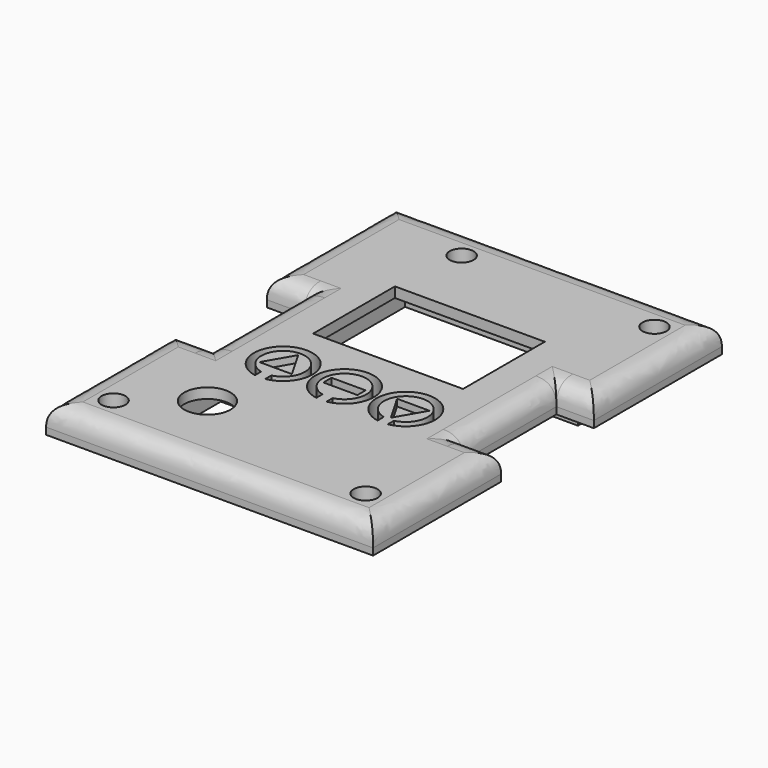
from build123d import *

# Parameters (mm, degrees)
F0_W          = 48
F0_H          = 64
F1_DEPTH      = 4
F2_W          = 5.5
F2_H          = 17
F3_DEPTH      = 4
F5_DEPTH      = 1.5
F6_R          = 1.05
F7_DEPTH      = 4
F8_W          = 22
F8_H          = 15
F9_DEPTH      = 5.501
F10_R         = 3.4
F11_DEPTH     = 5.501
F13_DEPTH     = 5.501
F14_W         = 14
F14_H         = 3.5
F15_DEPTH     = 4
F16_W         = 5
F16_H         = 1.5
F17_DEPTH     = 1
F19_DEPTH     = 4
F21_DEPTH     = 5
F22_T1_DEPTH  = 63
F22_T3_DEPTH  = 38.5
F22_T5_DEPTH  = 13
F22_T7_DEPTH  = 17
F22_T9_DEPTH  = 38.5
F22_T11_DEPTH = 13
F22_T17_DEPTH = 24.5
F22_T21_DEPTH = 20.5
F22_T28_DEPTH = 20.5
F22_T32_DEPTH = 24.5
F22_T39_DEPTH = 20.5
F22_T43_DEPTH = 24.5
F22_T50_DEPTH = 24.5
F22_T54_DEPTH = 20.5
F23_R         = 1.75
F24_DEPTH     = 3


# Not quite as in the source:
# - a fillet or chamfer that OpenCascade refuses, or shapes differently, is made with other operations: its cross-section is extruded or revolved along the edge and cut away or added
# - a feature names something its author has since deleted; it is built from what else it names


with BuildPart() as f1:
    # F0 (on Top) → F1 (new body)
    with BuildSketch(Plane.XY):
        Rectangle(F0_W, F0_H)
    extrude(amount=F1_DEPTH)

    # F2 (on face) → F3 (cut, through all)
    with BuildSketch(Plane(origin=(0, 0, 0), x_dir=(1, 0, 0), z_dir=(0, 0, -1))):
        with Locations((-21.25, 0)):
            Rectangle(F2_W, F2_H)
        with Locations((21.25, 0)):
            Rectangle(F2_W, F2_H)
    extrude(amount=-F3_DEPTH, mode=Mode.SUBTRACT)

    # F4 (on face) → F5 (join)
    with BuildSketch(Plane(origin=(0, 0, 0), x_dir=(1, 0, 0), z_dir=(0, 0, -1))):
        Polygon((-20.4, -10.1), (-20.4, -28.4), (-11.9, -28.4), (-11.9, -24.3), (-7.7, -24.3), (-7.7, -28.4), (16.3, -28.4), (16.3, -24.3), (20.4, -24.3), (20.4, -10.1), (15.5, -10.1), (15.5, 10.1), (20.4, 10.1), (20.4, 24.3), (16.3, 24.3), (16.3, 28.4), (-16.3, 28.4), (-16.3, 24.3), (-20.4, 24.3), (-20.4, 10.1), (-15.5, 10.1), (-15.5, -10.1), align=None)
    extrude(amount=F5_DEPTH)

    # F6 (on face) → F7 (cut, through all)
    with BuildSketch(Plane(origin=(0, 0, 0), x_dir=(1, 0, 0), z_dir=(0, 0, -1))):
        with Locations((-9.8, -26.5)):
            Circle(F6_R)
        with Locations((18.5, -26.5)):
            Circle(F6_R)
        with Locations((18.5, 26.5)):
            Circle(F6_R)
        with Locations((-18.5, 26.5)):
            Circle(F6_R)
    extrude(amount=-F7_DEPTH, mode=Mode.SUBTRACT)

    # F8 (on face) → F9 (cut, through all)
    with BuildSketch(Plane(origin=(0, 0, -1.5), x_dir=(1, 0, 0), z_dir=(0, 0, -1))):
        with Locations((0, -8.25)):
            Rectangle(F8_W, F8_H)
    extrude(amount=-F9_DEPTH, mode=Mode.SUBTRACT)

    # F10 (on face) → F11 (cut, through all)
    with BuildSketch(Plane(origin=(0, 0, -1.5), x_dir=(1, 0, 0), z_dir=(0, 0, -1))):
        with Locations((-10, 19.9)):
            Circle(F10_R)
    extrude(amount=-F11_DEPTH, mode=Mode.SUBTRACT)

    # F12 (on face) → F13 (cut, through all)
    with BuildSketch(Plane.XY.offset(4)):
        with BuildLine():
            ThreePointArc((0.75, -11.4840878593), (0, -2.95), (-0.75, -11.4840878593))
            Line((-0.75, -11.4840878593), (-0.75, -10.3608680461))
            ThreePointArc((-0.75, -10.3608680461), (0, -4.05), (0.75, -10.3608680461))
            Line((0.75, -10.3608680461), (0.75, -11.4840878593))
        make_face()
        with BuildLine():
            ThreePointArc((9.75, -11.4840878593), (9, -2.95), (8.25, -11.4840878593))
            Line((8.25, -11.4840878593), (8.25, -10.3608680461))
            ThreePointArc((8.25, -10.3608680461), (9, -4.05), (9.75, -10.3608680461))
            Line((9.75, -10.3608680461), (9.75, -11.4840878593))
        make_face()
        with BuildLine():
            ThreePointArc((-8.25, -11.4840878593), (-9, -2.95), (-9.75, -11.4840878593))
            Line((-9.75, -11.4840878593), (-9.75, -10.3608680461))
            ThreePointArc((-9.75, -10.3608680461), (-9, -4.05), (-8.25, -10.3608680461))
            Line((-8.25, -10.3608680461), (-8.25, -11.4840878593))
        make_face()
    extrude(amount=-F13_DEPTH, mode=Mode.SUBTRACT)

    # F14 (on face) → F15 (cut)
    with BuildSketch(Plane(origin=(0, 0, -1.5), x_dir=(1, 0, 0), z_dir=(0, 0, -1))):
        Polygon((-7, -0.75), (-13.5, -0.75), (-13.5, -20.75), (13.5, -20.75), (13.5, -0.75), (7, -0.75), align=None)
        with Locations((0, 1)):
            Rectangle(F14_W, F14_H)
    extrude(amount=-F15_DEPTH, mode=Mode.SUBTRACT)

    # F16 (on face) → F17 (cut)
    with BuildSketch(Plane.XY.offset(4)):
        Polygon((11.3815698604, -5.875), (6.6184301396, -5.875), (9, -10), align=None)
        Polygon((-9, -4.5), (-11.3815698604, -8.625), (-6.6184301396, -8.625), align=None)
        with Locations((0, -7.25)):
            Rectangle(F16_W, F16_H)
    extrude(amount=-F17_DEPTH, mode=Mode.SUBTRACT)

    # F18 (on face) → F19 (cut)
    with BuildSketch(Plane(origin=(0, 0, -1.5), x_dir=(1, 0, 0), z_dir=(0, 0, -1))):
        with BuildLine():
            ThreePointArc((-11.4264171117, 10.8), (-11.0070384176, 3.4471330828), (-4.7, 7.25))
            ThreePointArc((-4.7, 7.25), (-5.1971330828, 9.2570384176), (-6.5735828883, 10.8))
            Line((-6.5735828883, 10.8), (-11.4264171117, 10.8))
        make_face()
        with BuildLine():
            Line((-11.4264171117, 10.8), (-6.5735828883, 10.8))
            ThreePointArc((-6.5735828883, 10.8), (-9, 11.55), (-11.4264171117, 10.8))
        make_face()
        with BuildLine():
            ThreePointArc((-11.4264171117, 10.8), (-9, 11.55), (-6.5735828883, 10.8))
            Line((-6.5735828883, 10.8), (-2.4264171117, 10.8))
            ThreePointArc((-2.4264171117, 10.8), (0, 11.55), (2.4264171117, 10.8))
            Line((2.4264171117, 10.8), (6.5735828883, 10.8))
            ThreePointArc((6.5735828883, 10.8), (9, 11.55), (11.4264171117, 10.8))
            Line((11.4264171117, 10.8), (15.2, 10.8))
            Line((15.2, 10.8), (15.2, 26.3))
            Line((15.2, 26.3), (-15.3, 26.3))
            Line((-15.3, 26.3), (-15.3, 10.8))
            Line((-15.3, 10.8), (-11.4264171117, 10.8))
        make_face()
        with BuildLine():
            Line((2.4264171117, 10.8), (-2.4264171117, 10.8))
            ThreePointArc((-2.4264171117, 10.8), (-2.0070384176, 3.4471330828), (4.3, 7.25))
            ThreePointArc((4.3, 7.25), (3.8028669172, 9.2570384176), (2.4264171117, 10.8))
        make_face()
        with BuildLine():
            ThreePointArc((2.4264171117, 10.8), (0, 11.55), (-2.4264171117, 10.8))
            Line((-2.4264171117, 10.8), (2.4264171117, 10.8))
        make_face()
        with BuildLine():
            Line((11.4264171117, 10.8), (6.5735828883, 10.8))
            ThreePointArc((6.5735828883, 10.8), (6.9929615824, 3.4471330828), (13.3, 7.25))
            ThreePointArc((13.3, 7.25), (12.8028669172, 9.2570384176), (11.4264171117, 10.8))
        make_face()
        with BuildLine():
            ThreePointArc((11.4264171117, 10.8), (9, 11.55), (6.5735828883, 10.8))
            Line((6.5735828883, 10.8), (11.4264171117, 10.8))
        make_face()
    extrude(amount=-F19_DEPTH, mode=Mode.SUBTRACT)

    # F20 (on face) → F21 (join)
    with BuildSketch(Plane(origin=(0, 0, 2.5), x_dir=(1, 0, 0), z_dir=(0, 0, -1))):
        Polygon((6.6184301396, 5.875), (11.3815698604, 5.875), (9, 10), align=None)
        Polygon((-2.3815698604, 5.875), (2.3815698604, 5.875), (0, 10), align=None)
        Polygon((-11.3815698604, 5.875), (-6.6184301396, 5.875), (-9, 10), align=None)
    extrude(amount=F21_DEPTH)

    # F22: fillet of radius 3 on 12 edges, made by hand

    # F22_s2 → F22_t1 (cut)
    with BuildSketch(Plane.YZ.offset(-31.5)):
        with BuildLine():
            add(Edge.make_bspline(
                [(-29, 4), (-32, 4), (-32, 1)],
                knots=[0, 0, 0, 1, 1, 1], degree=2, weights=[1, 1, 1]))
            Line((-32, 1), (-32, 4))
            Line((-32, 4), (-29, 4))
        make_face()
        with BuildLine():
            add(Edge.make_bspline(
                [(32, 1), (32, 4), (29, 4)],
                knots=[0, 0, 0, 1, 1, 1], degree=2, weights=[1, 1, 1]))
            Line((29, 4), (32, 4))
            Line((32, 4), (32, 1))
        make_face()
    extrude(amount=F22_T1_DEPTH, mode=Mode.SUBTRACT)

    # F22_s4 → F22_t3 (cut)
    with BuildSketch(Plane.XZ.offset(1)):
        with BuildLine():
            add(Edge.make_bspline(
                [(21, 4), (24, 4), (24, 1)],
                knots=[0, 0, 0, 1, 1, 1], degree=2, weights=[1, 1, 1]))
            Line((24, 1), (24, 4))
            Line((24, 4), (21, 4))
        make_face()
        with BuildLine():
            add(Edge.make_bspline(
                [(-21, 4), (-24, 4), (-24, 1)],
                knots=[0, 0, 0, 1, 1, 1], degree=2, weights=[1, 1, 1]))
            Line((-24, 1), (-24, 4))
            Line((-24, 4), (-21, 4))
        make_face()
    extrude(amount=F22_T3_DEPTH, mode=Mode.SUBTRACT)

    # F22_s6 → F22_t5 (cut)
    with BuildSketch(Plane.YZ.offset(18.5)):
        with BuildLine():
            add(Edge.make_bspline(
                [(-11.5, 4), (-8.5, 4), (-8.5, 1)],
                knots=[0, 0, 0, 1, 1, 1], degree=2, weights=[1, 1, 1]))
            Line((-8.5, 1), (-8.5, 4))
            Line((-8.5, 4), (-11.5, 4))
        make_face()
        with BuildLine():
            add(Edge.make_bspline(
                [(11.5, 4), (8.5, 4), (8.5, 1)],
                knots=[0, 0, 0, 1, 1, 1], degree=2, weights=[1, 1, 1]))
            Line((8.5, 1), (8.5, 4))
            Line((8.5, 4), (11.5, 4))
        make_face()
    extrude(amount=F22_T5_DEPTH, mode=Mode.SUBTRACT)

    # F22_s8 → F22_t7 (cut)
    with BuildSketch(Plane.XZ.offset(-8.5)):
        with BuildLine():
            add(Edge.make_bspline(
                [(15.5, 4), (18.5, 4), (18.5, 1)],
                knots=[0, 0, 0, 1, 1, 1], degree=2, weights=[1, 1, 1]))
            Line((18.5, 1), (18.5, 4))
            Line((18.5, 4), (15.5, 4))
        make_face()
        with BuildLine():
            add(Edge.make_bspline(
                [(-15.5, 4), (-18.5, 4), (-18.5, 1)],
                knots=[0, 0, 0, 1, 1, 1], degree=2, weights=[1, 1, 1]))
            Line((-18.5, 1), (-18.5, 4))
            Line((-18.5, 4), (-15.5, 4))
        make_face()
    extrude(amount=F22_T7_DEPTH, mode=Mode.SUBTRACT)

    # F22_s10 → F22_t9 (cut)
    with BuildSketch(Plane.XZ.offset(-39.5)):
        with BuildLine():
            add(Edge.make_bspline(
                [(24, 1), (24, 4), (21, 4)],
                knots=[0, 0, 0, 1, 1, 1], degree=2, weights=[1, 1, 1]))
            Line((21, 4), (24, 4))
            Line((24, 4), (24, 1))
        make_face()
        with BuildLine():
            add(Edge.make_bspline(
                [(-24, 1), (-24, 4), (-21, 4)],
                knots=[0, 0, 0, 1, 1, 1], degree=2, weights=[1, 1, 1]))
            Line((-21, 4), (-24, 4))
            Line((-24, 4), (-24, 1))
        make_face()
    extrude(amount=F22_T9_DEPTH, mode=Mode.SUBTRACT)

    # F22_s12 → F22_t11 (cut)
    with BuildSketch(Plane.YZ.offset(-31.5)):
        with BuildLine():
            add(Edge.make_bspline(
                [(11.5, 4), (8.5, 4), (8.5, 1)],
                knots=[0, 0, 0, 1, 1, 1], degree=2, weights=[1, 1, 1]))
            Line((8.5, 1), (8.5, 4))
            Line((8.5, 4), (11.5, 4))
        make_face()
        with BuildLine():
            add(Edge.make_bspline(
                [(-11.5, 4), (-8.5, 4), (-8.5, 1)],
                knots=[0, 0, 0, 1, 1, 1], degree=2, weights=[1, 1, 1]))
            Line((-8.5, 1), (-8.5, 4))
            Line((-8.5, 4), (-11.5, 4))
        make_face()
    extrude(amount=F22_T11_DEPTH, mode=Mode.SUBTRACT)


with BuildPart() as f22_tool15:
    # F22_s16 → F22_t17 (new body)
    with BuildSketch(Plane.XZ.offset(16)):
        with BuildLine():
            add(Edge.make_bspline(
                [(15.5, 4), (18.5, 4), (18.5, 1)],
                knots=[0, 0, 0, 1, 1, 1], degree=2, weights=[1, 1, 1]))
            Line((18.5, 1), (18.5, 4))
            Line((18.5, 4), (15.5, 4))
        make_face()
    extrude(amount=-F22_T17_DEPTH)

    split(bisect_by=Plane.XZ.offset(8.5), keep=Keep.TOP)


with BuildPart() as f22_tool19:
    # F22_s20 → F22_t21 (new body)
    with BuildSketch(Plane.YZ.offset(31.5)):
        with BuildLine():
            add(Edge.make_bspline(
                [(-11.5, 4), (-8.5, 4), (-8.5, 1)],
                knots=[0, 0, 0, 1, 1, 1], degree=2, weights=[1, 1, 1]))
            Line((-8.5, 1), (-8.5, 4))
            Line((-8.5, 4), (-11.5, 4))
        make_face()
    extrude(amount=-F22_T21_DEPTH)

    split(bisect_by=Plane.YZ.offset(18.5), keep=Keep.BOTTOM)


with BuildPart() as f22_tool15_1:
    add(f22_tool15.part)

    # F22_t23: intersect F22_tool19
    add(f22_tool19.part, mode=Mode.INTERSECT)


with BuildPart() as f1_1:
    add(f1.part)

    # F22_t13: cut F22_tool15
    add(f22_tool15_1.part, mode=Mode.SUBTRACT)


with BuildPart() as f22_tool26:
    # F22_s27 → F22_t28 (new body)
    with BuildSketch(Plane.YZ.offset(11)):
        with BuildLine():
            add(Edge.make_bspline(
                [(11.5, 4), (8.5, 4), (8.5, 1)],
                knots=[0, 0, 0, 1, 1, 1], degree=2, weights=[1, 1, 1]))
            Line((8.5, 1), (8.5, 4))
            Line((8.5, 4), (11.5, 4))
        make_face()
    extrude(amount=F22_T28_DEPTH)

    split(bisect_by=Plane.YZ.offset(18.5), keep=Keep.BOTTOM)


with BuildPart() as f22_tool30:
    # F22_s31 → F22_t32 (new body)
    with BuildSketch(Plane.XZ.offset(8.5)):
        with BuildLine():
            add(Edge.make_bspline(
                [(15.5, 4), (18.5, 4), (18.5, 1)],
                knots=[0, 0, 0, 1, 1, 1], degree=2, weights=[1, 1, 1]))
            Line((18.5, 1), (18.5, 4))
            Line((18.5, 4), (15.5, 4))
        make_face()
    extrude(amount=-F22_T32_DEPTH)

    split(bisect_by=Plane.XZ.offset(-8.5), keep=Keep.BOTTOM)


with BuildPart() as f22_tool26_1:
    add(f22_tool26.part)

    # F22_t34: intersect F22_tool30
    add(f22_tool30.part, mode=Mode.INTERSECT)


with BuildPart() as f1_2:
    add(f1_1.part)

    # F22_t24: cut F22_tool26
    add(f22_tool26_1.part, mode=Mode.SUBTRACT)


with BuildPart() as f22_tool37:
    # F22_s38 → F22_t39 (new body)
    with BuildSketch(Plane.YZ.offset(-31.5)):
        with BuildLine():
            add(Edge.make_bspline(
                [(11.5, 4), (8.5, 4), (8.5, 1)],
                knots=[0, 0, 0, 1, 1, 1], degree=2, weights=[1, 1, 1]))
            Line((8.5, 1), (8.5, 4))
            Line((8.5, 4), (11.5, 4))
        make_face()
    extrude(amount=F22_T39_DEPTH)

    split(bisect_by=Plane.YZ.offset(-18.5), keep=Keep.TOP)


with BuildPart() as f22_tool41:
    # F22_s42 → F22_t43 (new body)
    with BuildSketch(Plane.XZ.offset(-16)):
        with BuildLine():
            add(Edge.make_bspline(
                [(-15.5, 4), (-18.5, 4), (-18.5, 1)],
                knots=[0, 0, 0, 1, 1, 1], degree=2, weights=[1, 1, 1]))
            Line((-18.5, 1), (-18.5, 4))
            Line((-18.5, 4), (-15.5, 4))
        make_face()
    extrude(amount=F22_T43_DEPTH)

    split(bisect_by=Plane.XZ.offset(-8.5), keep=Keep.BOTTOM)


with BuildPart() as f22_tool37_1:
    add(f22_tool37.part)

    # F22_t45: intersect F22_tool41
    add(f22_tool41.part, mode=Mode.INTERSECT)


with BuildPart() as f1_3:
    add(f1_2.part)

    # F22_t35: cut F22_tool37
    add(f22_tool37_1.part, mode=Mode.SUBTRACT)


with BuildPart() as f22_tool48:
    # F22_s49 → F22_t50 (new body)
    with BuildSketch(Plane.XZ.offset(-8.5)):
        with BuildLine():
            add(Edge.make_bspline(
                [(-15.5, 4), (-18.5, 4), (-18.5, 1)],
                knots=[0, 0, 0, 1, 1, 1], degree=2, weights=[1, 1, 1]))
            Line((-18.5, 1), (-18.5, 4))
            Line((-18.5, 4), (-15.5, 4))
        make_face()
    extrude(amount=F22_T50_DEPTH)

    split(bisect_by=Plane.XZ.offset(8.5), keep=Keep.TOP)


with BuildPart() as f22_tool52:
    # F22_s53 → F22_t54 (new body)
    with BuildSketch(Plane.YZ.offset(-11)):
        with BuildLine():
            add(Edge.make_bspline(
                [(-11.5, 4), (-8.5, 4), (-8.5, 1)],
                knots=[0, 0, 0, 1, 1, 1], degree=2, weights=[1, 1, 1]))
            Line((-8.5, 1), (-8.5, 4))
            Line((-8.5, 4), (-11.5, 4))
        make_face()
    extrude(amount=-F22_T54_DEPTH)

    split(bisect_by=Plane.YZ.offset(-18.5), keep=Keep.TOP)


with BuildPart() as f22_tool48_1:
    add(f22_tool48.part)

    # F22_t56: intersect F22_tool52
    add(f22_tool52.part, mode=Mode.INTERSECT)


with BuildPart() as f1_4:
    add(f1_3.part)

    # F22_t46: cut F22_tool48
    add(f22_tool48_1.part, mode=Mode.SUBTRACT)

    # F23 (on face) → F24 (cut)
    with BuildSketch(Plane.XY.offset(4)):
        with Locations((-9.8, 26.5)):
            Circle(F23_R)
        with Locations((18.5, 26.5)):
            Circle(F23_R)
        with Locations((-18.5, -26.5)):
            Circle(F23_R)
        with Locations((18.5, -26.5)):
            Circle(F23_R)
    extrude(amount=-F24_DEPTH, mode=Mode.SUBTRACT)


solid = f1_4.part
